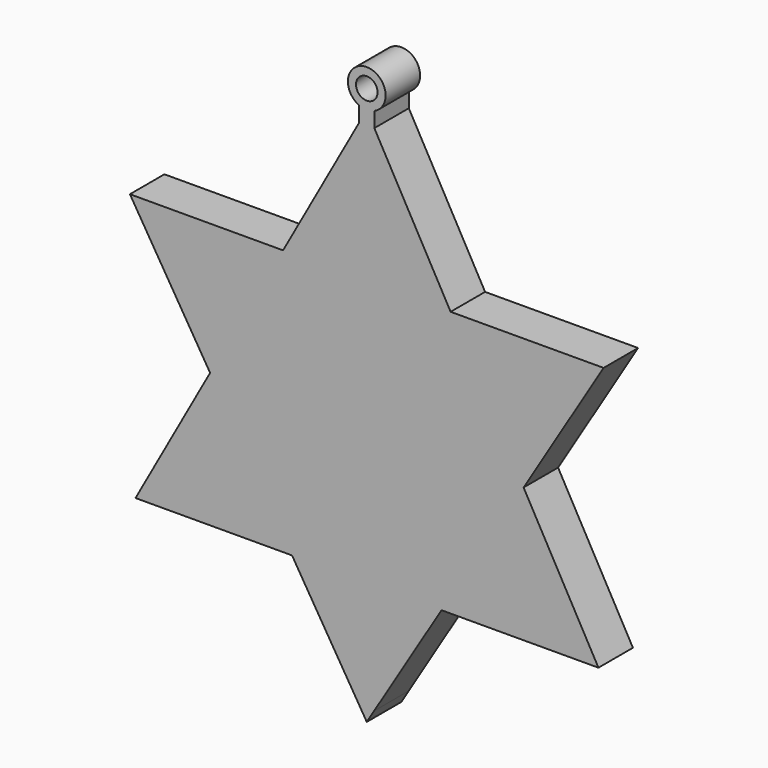
from build123d import *

# Parameters (mm, degrees)
F0_R         = 2
F1_DEPTH     = 8
F2_TEXT_SIZE = 11.1111111111
F3_DEPTH     = 1.5


# Not quite as in the source:
# - Text() gives the source's letters only with a copy of the font that has no kerning and outlines rounded to 1/6400 em; it was checked with that copy


with BuildPart() as f1:
    # F0 (on Front) → F1 (new body)
    with BuildSketch(Plane.XZ):
        with BuildLine():
            Line((-15.5314165364, 24.6576191819), (-43.9586468074, 24.5899649613))
            Line((-43.9586468074, 24.5899649613), (-29.0768258474, 0.237916982))
            Line((-29.0768258474, 0.237916982), (-42.9202532426, -24.719053063))
            Line((-42.9202532426, -24.719053063), (-13.8703300812, -24.645416549))
            Line((-13.8703300812, -24.645416549), (-1.3718173327, -45.0975092692))
            Line((-1.3718173327, -45.0975092692), (0, -47.3422991773))
            Line((0, -47.3422991773), (1.3718173327, -45.0909796684))
            Line((1.3718173327, -45.0909796684), (13.8729527756, -24.5750921413))
            Line((13.8729527756, -24.5750921413), (43.00164739, -24.5012559553))
            Line((43.00164739, -24.5012559553), (29.1082891257, 0.427952456))
            Line((29.1082891257, 0.427952456), (43.9586468074, 24.799200118))
            Line((43.9586468074, 24.799200118), (15.5635512523, 24.7316223751))
            Line((15.5635512523, 24.7316223751), (1.4051777792, 50.1363543602))
            Line((1.4051777792, 50.1363543602), (1.4051777792, 52.9521625826))
            ThreePointArc((1.4051777792, 52.9521625826), (0, 59.6577008227), (-1.4051777792, 52.9521625826))
            Line((-1.4051777792, 52.9521625826), (-1.4051777792, 50.1244423498))
            Line((-1.4051777792, 50.1244423498), (-15.5314165364, 24.6576191819))
        make_face()
        with Locations((0, 56.1577008227)):
            Circle(F0_R, mode=Mode.SUBTRACT)
    extrude(amount=F1_DEPTH)

    # F2 (on face) → F3 (join)
    with BuildSketch(Plane(origin=(0, 0, 0), x_dir=(-1, 0, 0), z_dir=(0, 1, 0))):
        with Locations((-20.826276215, 12.4287227243)):
            Text('HOPE &', F2_TEXT_SIZE, font='Open Sans', text_align=(TextAlign.LEFT, TextAlign.BOTTOM))
        with Locations((-17.9391234372, -2.6823883868)):
            Text('CHRIS', F2_TEXT_SIZE, font='Open Sans', text_align=(TextAlign.LEFT, TextAlign.BOTTOM))
        with Locations((-23.7134289928, -17.7934994979)):
            Text("XMAS '15", F2_TEXT_SIZE, font='Open Sans', text_align=(TextAlign.LEFT, TextAlign.BOTTOM))
    extrude(amount=F3_DEPTH)


solid = f1.part
